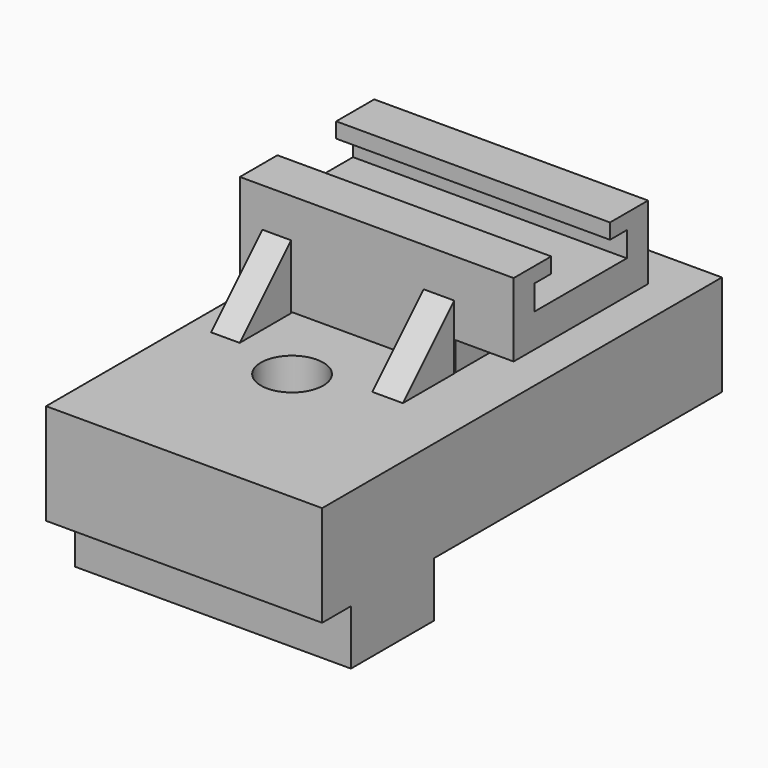
from build123d import *

# Parameters (mm, degrees)
F1_DEPTH    = 84.328
F2_W        = 8.7442607619
F2_H        = 19.8203269392
F2_W_2      = 9.3272216618
F3_DEPTH    = 25.4
F4_T4_DEPTH = 139.3857565506
F4_T9_DEPTH = 139.9687174505
F5_R        = 9.525
F6_DEPTH    = 36.83
F8_DEPTH    = 51.308
F10_DEPTH   = 88.9


# Not quite as in the source:
# - a fillet or chamfer that OpenCascade refuses, or shapes differently, is made with other operations: its cross-section is extruded or revolved along the edge and cut away or added


with BuildPart() as f1:
    # F0 (on Right) → F1 (new body)
    with BuildSketch(Plane.YZ):
        Polygon((78.6539154417, 24.2497121325), (-73.9903064734, 24.2497121325), (-73.9903064734, -6.584421545), (-62.9999262101, -6.584421545), (-62.9999262101, -23.3752859166), (-31.2499262101, -23.3752859166), (-31.2499262101, -6.584421545), (78.6539154417, -6.584421545), align=None)
    extrude(amount=F1_DEPTH)

    # F2 (on Front) → F3 (join)
    with BuildSketch(Plane.XZ):
        with Locations((11.2704045605, 33.9568844065)):
            Rectangle(F2_W, F2_H)
        with Locations((60.8212258667, 33.9568844065)):
            Rectangle(F2_W_2, F2_H)
    extrude(amount=F3_DEPTH)

    # F4: chamfer of 25.4 on 2 edges, made by hand


with BuildPart() as f4_tool2:
    # F4_s3 → F4_t4 (new body)
    with BuildSketch(Plane.YZ.offset(80.9632828358)):
        Polygon((-25.4, 18.4670478761), (0, 43.8670478761), (-25.4, 43.8670478761), align=None)
    extrude(amount=-F4_T4_DEPTH)

    split(bisect_by=Plane.XY.offset(24.2497121325), keep=Keep.TOP)


with BuildPart() as f1_1:
    add(f1.part)

    # F4_t1: cut F4_tool2
    add(f4_tool2.part, mode=Mode.SUBTRACT)


with BuildPart() as f4_tool7:
    # F4_s8 → F4_t9 (new body)
    with BuildSketch(Plane.YZ.offset(130.8055845919)):
        Polygon((-25.4, 18.4670478761), (0, 43.8670478761), (-25.4, 43.8670478761), align=None)
    extrude(amount=-F4_T9_DEPTH)

    split(bisect_by=Plane.XY.offset(24.2497121325), keep=Keep.TOP)


with BuildPart() as f1_2:
    add(f1_1.part)

    # F4_t6: cut F4_tool7
    add(f4_tool7.part, mode=Mode.SUBTRACT)

    # F5 (on Top) → F6 (cut)
    with BuildSketch(Plane.XY):
        with Locations((35.4578830302, -24.3916343898)):
            Circle(F5_R)
    extrude(amount=F6_DEPTH, mode=Mode.SUBTRACT)

    # F7 (on Front) → F8 (join)
    with BuildSketch(Plane.XZ):
        Polygon((65.8567920327, 24.6296729892), (65.8567920327, 33.3739332855), (83.636790514, 33.3739332855), (83.636790514, 55.8175444603), (0, 55.8175444603), (0, 24.6296729892), align=None)
    extrude(amount=-F8_DEPTH)

    # F9 (on Right) → F10 (cut)
    with BuildSketch(Plane.YZ):
        Polygon((36.7869585752, 56.1090186238), (14.3433511257, 56.1090186238), (14.3433511257, 51.153935492), (7.930893451, 51.153935492), (7.930893451, 43.5755737126), (43.1994171752, 43.5755737126), (43.1994171752, 51.153935492), (36.7869585752, 51.153935492), align=None)
    extrude(amount=F10_DEPTH, mode=Mode.SUBTRACT)


solid = f1_2.part
